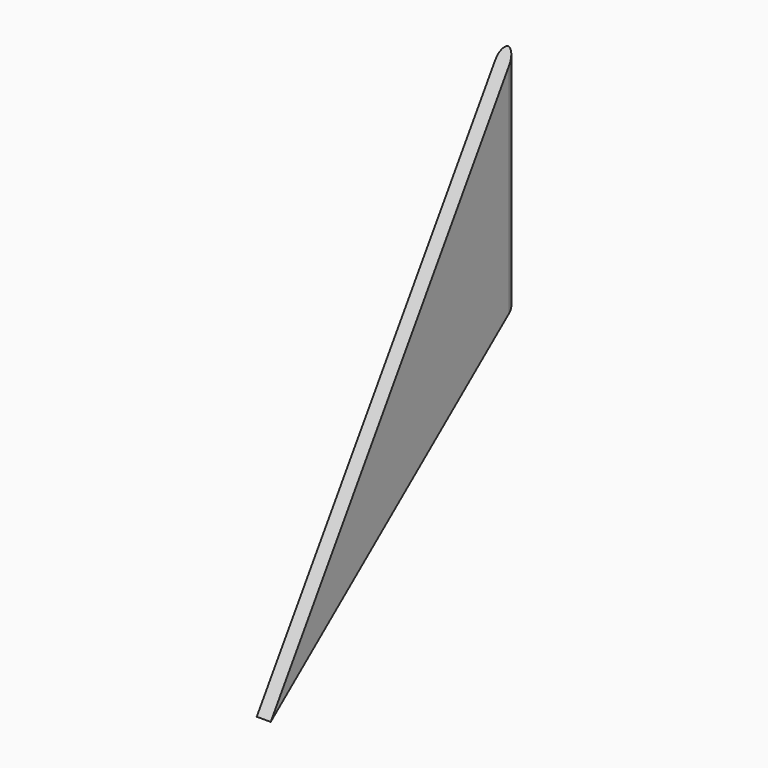
from build123d import *

# Parameters (mm, degrees)
F1_DEPTH    = 2.5
F2_T1_DEPTH = 46.75


# Not quite as in the source:
# - a fillet or chamfer that OpenCascade refuses, or shapes differently, is made with other operations: its cross-section is extruded or revolved along the edge and cut away or added


with BuildPart() as f1:
    # F0 (on Right) → F1 (new body)
    with BuildSketch(Plane.YZ):
        Polygon((-54.643732486, -43.75), (0, 0), (0, 40), align=None)
    extrude(amount=F1_DEPTH)

    # F2: fillet of radius 1.35 on 2 edges, made by hand

    # F2_s2 → F2_t1 (cut)
    with BuildSketch(Plane.XY.offset(-3.375)):
        with BuildLine():
            ThreePointArc((1.15, 0), (2.1045941546, -0.3954058454), (2.5, -1.35))
            Line((2.5, -1.35), (2.5, 0))
            Line((2.5, 0), (1.15, 0))
        make_face()
        with BuildLine():
            ThreePointArc((1.35, 0), (0.3954058454, -0.3954058454), (0, -1.35))
            Line((0, -1.35), (0, 0))
            Line((0, 0), (1.35, 0))
        make_face()
    extrude(amount=F2_T1_DEPTH, mode=Mode.SUBTRACT)


solid = f1.part
